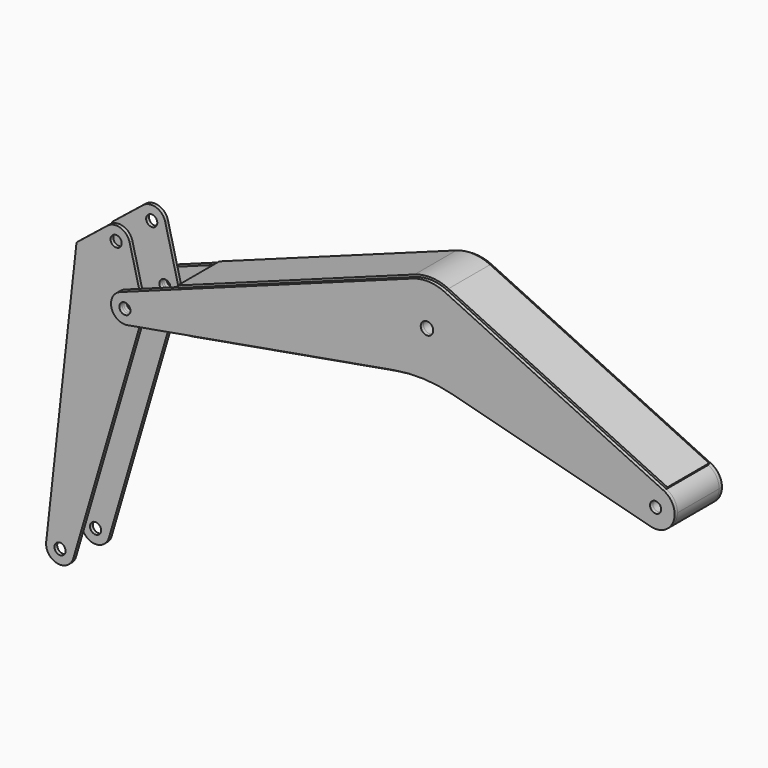
from build123d import *

# Parameters (mm, degrees)
F0_R      = 17.5
F0_R_2    = 8
F1_DEPTH  = 5
F0_R_3    = 15
F0_R_4    = 22.5
F0_R_5    = 9
F2_DEPTH  = 5
F4_R      = 17.5
F4_R_2    = 22.5
F4_R_3    = 9
F4_R_4    = 8
F5_DEPTH  = 5
F6_DEPTH  = 75
F7_DEPTH  = 75
F9_DEPTH  = 75
F10_DEPTH = 75
F11_DEPTH = 75
F8_R      = 17.5
F12_DEPTH = 3
F14_DEPTH = 3
F16_R     = 17.5
F16_R_2   = 8
F17_DEPTH = 5
F19_R     = 17.5
F19_R_2   = 8
F20_DEPTH = 5


# Not quite as in the source:
# - a feature names something its author has since deleted; it is built from what else it names


with BuildPart() as f1:
    # F0 (on Front) → F1 (new body)
    with BuildSketch(Plane.XZ):
        with Locations((-434.6666218301, -116.4685702961)):
            Circle(F0_R)
        with Locations((-434.6666218301, -116.4685702961)):
            Circle(F0_R_2, mode=Mode.SUBTRACT)
    extrude(amount=F1_DEPTH)


with BuildPart() as f2:
    # F0 (on Front) → F2 (new body)
    with BuildSketch(Plane.XZ):
        with BuildLine():
            ThreePointArc((25.6679758413, 54.2324166547), (50.6955547878, 32.0930011803), (60, 0))
            ThreePointArc((60, 0), (-34.3718158899, -49.1790430207), (-20.6192757477, 56.3457670783))
            Line((-20.6192757477, 56.3457670783), (-441.539713746, -97.6866479367))
            ThreePointArc((-441.539713746, -97.6866479367), (-423.2093498668, -100.0755559559), (-414.6666218301, -116.4685702961))
            ThreePointArc((-414.6666218301, -116.4685702961), (-419.3438009709, -129.3220196743), (-431.1877379217, -136.1636805206))
            Line((-431.1877379217, -136.1636805206), (-47.6857460535, -68.4230640354))
            ThreePointArc((-47.6857460535, -68.4230640354), (-4.8047190164, -65.5411431254), (37.7010021837, -71.8934350856))
            Line((37.7010021837, -71.8934350856), (321.927072804, -146.310320196))
            ThreePointArc((321.927072804, -146.310320196), (303.0508702035, -110.3014962225), (340.6569062023, -94.8505258639))
            Line((340.6569062023, -94.8505258639), (25.6679758413, 54.2324166547))
        make_face()
        with BuildLine():
            ThreePointArc((-20.6192757477, 56.3457670783), (-34.3718158899, -49.1790430207), (60, 0))
            ThreePointArc((60, 0), (50.6955547878, 32.0930011803), (25.6679758413, 54.2324166547))
            ThreePointArc((25.6679758413, 54.2324166547), (2.7365864982, 59.9375599632), (-20.6192757477, 56.3457670783))
        make_face()
        Circle(F0_R_3, mode=Mode.SUBTRACT)
        with BuildLine():
            ThreePointArc((356.3924172751, -119.707050164), (352.1278798861, -104.9977579563), (340.6569062023, -94.8505258639))
            ThreePointArc((340.6569062023, -94.8505258639), (303.0508702035, -110.3014962225), (321.927072804, -146.310320196))
            ThreePointArc((321.927072804, -146.310320196), (345.6957358021, -141.476259761), (356.3924172751, -119.707050164))
        make_face()
        with Locations((328.8924172751, -119.707050164)):
            Circle(F0_R_4, mode=Mode.SUBTRACT)
        with Locations((328.8924172751, -119.707050164)):
            Circle(F0_R_4)
        with Locations((328.8924172751, -119.707050164)):
            Circle(F0_R_2, mode=Mode.SUBTRACT)
        with BuildLine():
            ThreePointArc((-414.6666218301, -116.4685702961), (-423.2093498668, -100.0755559559), (-441.539713746, -97.6866479367))
            ThreePointArc((-441.539713746, -97.6866479367), (-453.9798471204, -121.6646581405), (-431.1877379217, -136.1636805206))
            ThreePointArc((-431.1877379217, -136.1636805206), (-419.3438009709, -129.3220196743), (-414.6666218301, -116.4685702961))
        make_face()
        with Locations((-434.6666218301, -116.4685702961)):
            Circle(F0_R, mode=Mode.SUBTRACT)
        with Locations((-434.6666218301, -116.4685702961)):
            Circle(F0_R)
        with Locations((-434.6666218301, -116.4685702961)):
            Circle(F0_R_2, mode=Mode.SUBTRACT)
        Circle(F0_R_3)
        Circle(F0_R_5, mode=Mode.SUBTRACT)
        Circle(F0_R_5)
        Circle(F0_R_2, mode=Mode.SUBTRACT)
    extrude(amount=-F2_DEPTH)


with BuildPart() as f5:
    # F4 (on offset) → F5 (new body)
    with BuildSketch(Plane.XZ.offset(75)):
        with BuildLine():
            Line((340.6569062023, -94.8505258639), (25.6679758413, 54.2324166547))
            ThreePointArc((25.6679758413, 54.2324166547), (2.7365864982, 59.9375599632), (-20.6192757477, 56.3457670783))
            Line((-20.6192757477, 56.3457670783), (-441.539713746, -97.6866479367))
            ThreePointArc((-441.539713746, -97.6866479367), (-453.9798471204, -121.6646581405), (-431.1877379217, -136.1636805206))
            Line((-431.1877379217, -136.1636805206), (-47.6857460535, -68.4230640354))
            ThreePointArc((-47.6857460535, -68.4230640354), (-4.8047190164, -65.5411431254), (37.7010021837, -71.8934350856))
            Line((37.7010021837, -71.8934350856), (321.927072804, -146.310320196))
            ThreePointArc((321.927072804, -146.310320196), (354.7339643467, -129.1126041054), (340.6569062023, -94.8505258639))
        make_face()
        with Locations((-434.6666218301, -116.4685702961)):
            Circle(F4_R, mode=Mode.SUBTRACT)
        with Locations((328.8924172751, -119.707050164)):
            Circle(F4_R_2, mode=Mode.SUBTRACT)
        Circle(F4_R_3, mode=Mode.SUBTRACT)
        with Locations((328.8924172751, -119.707050164)):
            Circle(F4_R_2)
        with Locations((328.8924172751, -119.707050164)):
            Circle(F4_R_4, mode=Mode.SUBTRACT)
        with Locations((-434.6666218301, -116.4685702961)):
            Circle(F4_R)
        with Locations((-434.6666218301, -116.4685702961)):
            Circle(F4_R_4, mode=Mode.SUBTRACT)
    extrude(amount=F5_DEPTH)


with BuildPart() as f6:
    # F0 (on Front) → F6 (new body, through all)
    with BuildSketch(Plane.XZ):
        with BuildLine():
            ThreePointArc((356.3924172751, -119.707050164), (352.1278798861, -104.9977579563), (340.6569062023, -94.8505258639))
            ThreePointArc((340.6569062023, -94.8505258639), (303.0508702035, -110.3014962225), (321.927072804, -146.310320196))
            ThreePointArc((321.927072804, -146.310320196), (345.6957358021, -141.476259761), (356.3924172751, -119.707050164))
        make_face()
        with Locations((328.8924172751, -119.707050164)):
            Circle(F0_R_4, mode=Mode.SUBTRACT)
        with Locations((328.8924172751, -119.707050164)):
            Circle(F0_R_4)
        with Locations((328.8924172751, -119.707050164)):
            Circle(F0_R_2, mode=Mode.SUBTRACT)
    extrude(amount=F6_DEPTH)


with BuildPart() as f7:
    # F0 (on Front) → F7 (new body, through all)
    with BuildSketch(Plane.XZ):
        Circle(F0_R_3)
        Circle(F0_R_5, mode=Mode.SUBTRACT)
    extrude(amount=F7_DEPTH)


with BuildPart() as f9:
    # F8 (on face) → F9 (new body, through all)
    with BuildSketch(Plane.XZ.offset(75)):
        with BuildLine():
            Line((-361.7165437184, -68.4760072941), (-20.6192757477, 56.3457670783))
            ThreePointArc((-20.6192757477, 56.3457670783), (2.7365864982, 59.9375599632), (25.6679758413, 54.2324166547))
            Line((25.6679758413, 54.2324166547), (340.6569062023, -94.8505258639))
            Line((340.6569062023, -94.8505258639), (341.9403049944, -92.1389050312))
            Line((341.9403049944, -92.1389050312), (26.9513746334, 56.9440374875))
            ThreePointArc((26.9513746334, 56.9440374875), (2.8734158231, 62.9344379613), (-21.6502395351, 59.1630554322))
            Line((-21.6502395351, 59.1630554322), (-362.7475075058, -65.6587189402))
            Line((-362.7475075058, -65.6587189402), (-361.7165437184, -68.4760072941))
        make_face()
    extrude(amount=-F9_DEPTH)


with BuildPart() as f10:
    # F8 (on face) → F10 (new body, through all)
    with BuildSketch(Plane.XZ.offset(75)):
        with BuildLine():
            Line((321.1672170435, -149.2124951086), (321.927072804, -146.310320196))
            Line((321.927072804, -146.310320196), (37.7010021837, -71.8934350856))
            ThreePointArc((37.7010021837, -71.8934350856), (-4.8047190164, -65.5411431254), (-47.6857460535, -68.4230640354))
            Line((-47.6857460535, -68.4230640354), (-346.1877379217, -121.1495410289))
            Line((-346.1877379217, -121.1495410289), (-345.6659053354, -124.1038075626))
            Line((-345.6659053354, -124.1038075626), (-47.1639134672, -71.3773305691))
            ThreePointArc((-47.1639134672, -71.3773305691), (-4.9265473469, -68.5386684143), (36.9411464232, -74.7956099982))
            Line((36.9411464232, -74.7956099982), (321.1672170435, -149.2124951086))
        make_face()
    extrude(amount=-F10_DEPTH)


with BuildPart() as f11:
    # F8 (on face) → F11 (new body, through all)
    with BuildSketch(Plane.XZ.offset(75)):
        Polygon((-346.5125719091, -121.2069187089), (-361.9040511092, -68.5446241006), (-364.7208074131, -69.5753931886), (-349.4674006349, -121.728850599), align=None)
    extrude(amount=-F11_DEPTH)


with BuildPart() as f12:
    # F8 (on face) → F12 (new body)
    with BuildSketch(Plane.XZ.offset(75)):
        with BuildLine():
            Line((-349.4674006349, -121.728850599), (-364.7208074131, -69.5753931886))
            Line((-364.7208074131, -69.5753931886), (-441.539713746, -97.6866479367))
            ThreePointArc((-441.539713746, -97.6866479367), (-453.9798471204, -121.6646581405), (-431.1877379217, -136.1636805206))
            Line((-431.1877379217, -136.1636805206), (-349.4674006349, -121.728850599))
        make_face()
        with Locations((-434.6666218301, -116.4685702961)):
            Circle(F8_R, mode=Mode.SUBTRACT)
    extrude(amount=-F12_DEPTH)


with BuildPart() as f12b:
    # F4 (on offset) → F12, piece 2 (new body)
    with BuildSketch(Plane.XZ.offset(75)):
        with Locations((-434.6666218301, -116.4685702961)):
            Circle(F4_R)
        with Locations((-434.6666218301, -116.4685702961)):
            Circle(F4_R_4, mode=Mode.SUBTRACT)
    extrude(amount=-F12_DEPTH)


with BuildPart() as f14:
    # F13 (on face) → F14 (new body)
    with BuildSketch(Plane.XZ):
        with BuildLine():
            Line((-349.4674006349, -121.728850599), (-364.7208074131, -69.5753931886))
            Line((-364.7208074131, -69.5753931886), (-441.539713746, -97.6866479367))
            ThreePointArc((-441.539713746, -97.6866479367), (-423.2093498668, -100.0755559559), (-414.6666218301, -116.4685702961))
            ThreePointArc((-414.6666218301, -116.4685702961), (-419.3438009709, -129.3220196743), (-431.1877379217, -136.1636805206))
            Line((-431.1877379217, -136.1636805206), (-349.4674006349, -121.728850599))
        make_face()
    extrude(amount=F14_DEPTH)


with BuildPart() as f14b:
    # F0 (on Front) → F14, piece 2 (new body)
    with BuildSketch(Plane.XZ):
        with BuildLine():
            ThreePointArc((-414.6666218301, -116.4685702961), (-423.2093498668, -100.0755559559), (-441.539713746, -97.6866479367))
            ThreePointArc((-441.539713746, -97.6866479367), (-453.9798471204, -121.6646581405), (-431.1877379217, -136.1636805206))
            ThreePointArc((-431.1877379217, -136.1636805206), (-419.3438009709, -129.3220196743), (-414.6666218301, -116.4685702961))
        make_face()
        with Locations((-434.6666218301, -116.4685702961)):
            Circle(F0_R, mode=Mode.SUBTRACT)
        with Locations((-434.6666218301, -116.4685702961)):
            Circle(F0_R)
        with Locations((-434.6666218301, -116.4685702961)):
            Circle(F0_R_2, mode=Mode.SUBTRACT)
    extrude(amount=F14_DEPTH)


with BuildPart() as f17:
    # F16 (on offset) → F17 (new body)
    with BuildSketch(Plane(origin=(0, -72, 0), x_dir=(-1, 0, 0), z_dir=(0, 1, 0))):
        with BuildLine():
            ThreePointArc((415.476391148, -122.1019570545), (437.5122664283, -136.2650928903), (454.6666218301, -116.4685702961))
            ThreePointArc((454.6666218301, -116.4685702961), (437.110287104, -96.6184191625), (415.2637718272, -111.6178577954))
            ThreePointArc((415.2637718272, -111.6178577954), (414.670733415, -116.8740903231), (415.476391148, -122.1019570545))
        make_face()
        with Locations((434.6666218301, -116.4685702961)):
            Circle(F16_R, mode=Mode.SUBTRACT)
        with BuildLine():
            ThreePointArc((415.2637718272, -111.6178577954), (437.110287104, -96.6184191625), (454.6666218301, -116.4685702961))
            ThreePointArc((454.6666218301, -116.4685702961), (437.5122664283, -136.2650928903), (415.476391148, -122.1019570545))
            Line((415.476391148, -122.1019570545), (515.2850661759, -462.1019570545))
            ThreePointArc((515.2850661759, -462.1019570545), (530.5409299312, -436.8593694739), (554.3533493694, -454.26334279))
            Line((554.3533493694, -454.26334279), (510.6666218301, -60.4685702961))
            Line((510.6666218301, -60.4685702961), (466.163196234, -24.8533332449))
            ThreePointArc((466.163196234, -24.8533332449), (471.693428093, -31.8063387153), (473.6666218301, -40.4685702961))
            ThreePointArc((473.6666218301, -40.4685702961), (451.2229565562, -60.3187214298), (434.2637718272, -35.6178577954))
            Line((434.2637718272, -35.6178577954), (415.2637718272, -111.6178577954))
        make_face()
        with BuildLine():
            ThreePointArc((466.163196234, -24.8533332449), (447.2718655515, -21.5184491319), (434.2637718272, -35.6178577954))
            ThreePointArc((434.2637718272, -35.6178577954), (451.2229565562, -60.3187214298), (473.6666218301, -40.4685702961))
            ThreePointArc((473.6666218301, -40.4685702961), (471.693428093, -31.8063387153), (466.163196234, -24.8533332449))
        make_face()
        with Locations((453.6666218301, -40.4685702961)):
            Circle(F16_R_2, mode=Mode.SUBTRACT)
        with BuildLine():
            ThreePointArc((554.3533493694, -454.26334279), (530.5409299312, -436.8593694739), (515.2850661759, -462.1019570545))
            ThreePointArc((515.2850661759, -462.1019570545), (537.3209414562, -476.2650928903), (554.475296858, -456.4685702961))
            ThreePointArc((554.475296858, -456.4685702961), (554.4447867141, -455.364271928), (554.3533493694, -454.26334279))
        make_face()
        with Locations((534.475296858, -456.4685702961)):
            Circle(F16_R_2, mode=Mode.SUBTRACT)
        with Locations((434.6666218301, -116.4685702961)):
            Circle(F16_R)
        with Locations((434.6666218301, -116.4685702961)):
            Circle(F16_R_2, mode=Mode.SUBTRACT)
    extrude(amount=F17_DEPTH)


with BuildPart() as f20:
    # F19 (on face) → F20 (new body)
    with BuildSketch(Plane.XZ.offset(3)):
        with BuildLine():
            ThreePointArc((-415.476391148, -122.1019570545), (-414.8700992359, -119.3142148944), (-414.6666218301, -116.4685702961))
            ThreePointArc((-414.6666218301, -116.4685702961), (-414.8164706964, -114.0249050222), (-415.2637718272, -111.6178577954))
            ThreePointArc((-415.2637718272, -111.6178577954), (-454.6625102451, -116.0630502691), (-415.476391148, -122.1019570545))
        make_face()
        with Locations((-434.6666218301, -116.4685702961)):
            Circle(F19_R, mode=Mode.SUBTRACT)
        with BuildLine():
            ThreePointArc((-415.476391148, -122.1019570545), (-454.6625102451, -116.0630502691), (-415.2637718272, -111.6178577954))
            Line((-415.2637718272, -111.6178577954), (-434.2637718272, -35.6178577954))
            ThreePointArc((-434.2637718272, -35.6178577954), (-433.8164706964, -38.0249050222), (-433.6666218301, -40.4685702961))
            ThreePointArc((-433.6666218301, -40.4685702961), (-462.3288534109, -58.495376559), (-466.163196234, -24.8533332449))
            Line((-466.163196234, -24.8533332449), (-510.6666218301, -60.4685702961))
            Line((-510.6666218301, -60.4685702961), (-554.3533493694, -454.26334279))
            ThreePointArc((-554.3533493694, -454.26334279), (-533.3709984898, -436.49908044), (-514.475296858, -456.4685702961))
            ThreePointArc((-514.475296858, -456.4685702961), (-514.6787742638, -459.3142148944), (-515.2850661759, -462.1019570545))
            Line((-515.2850661759, -462.1019570545), (-415.476391148, -122.1019570545))
        make_face()
        with BuildLine():
            ThreePointArc((-433.6666218301, -40.4685702961), (-433.8164706964, -38.0249050222), (-434.2637718272, -35.6178577954))
            ThreePointArc((-434.2637718272, -35.6178577954), (-447.2718655515, -21.5184491319), (-466.163196234, -24.8533332449))
            ThreePointArc((-466.163196234, -24.8533332449), (-462.3288534109, -58.495376559), (-433.6666218301, -40.4685702961))
        make_face()
        with Locations((-453.6666218301, -40.4685702961)):
            Circle(F19_R_2, mode=Mode.SUBTRACT)
        with BuildLine():
            ThreePointArc((-554.3533493694, -454.26334279), (-538.4096637847, -476.0777711183), (-515.2850661759, -462.1019570545))
            ThreePointArc((-515.2850661759, -462.1019570545), (-514.6787742638, -459.3142148944), (-514.475296858, -456.4685702961))
            ThreePointArc((-514.475296858, -456.4685702961), (-533.3709984898, -436.49908044), (-554.3533493694, -454.26334279))
        make_face()
        with Locations((-534.475296858, -456.4685702961)):
            Circle(F19_R_2, mode=Mode.SUBTRACT)
        with Locations((-434.6666218301, -116.4685702961)):
            Circle(F19_R)
        with Locations((-434.6666218301, -116.4685702961)):
            Circle(F19_R_2, mode=Mode.SUBTRACT)
    extrude(amount=F20_DEPTH)


solid = Compound([f2.part, f5.part, f6.part, f7.part, f9.part, f10.part, f11.part, f12.part, f12b.part, f14.part, f14b.part, f17.part, f20.part])
